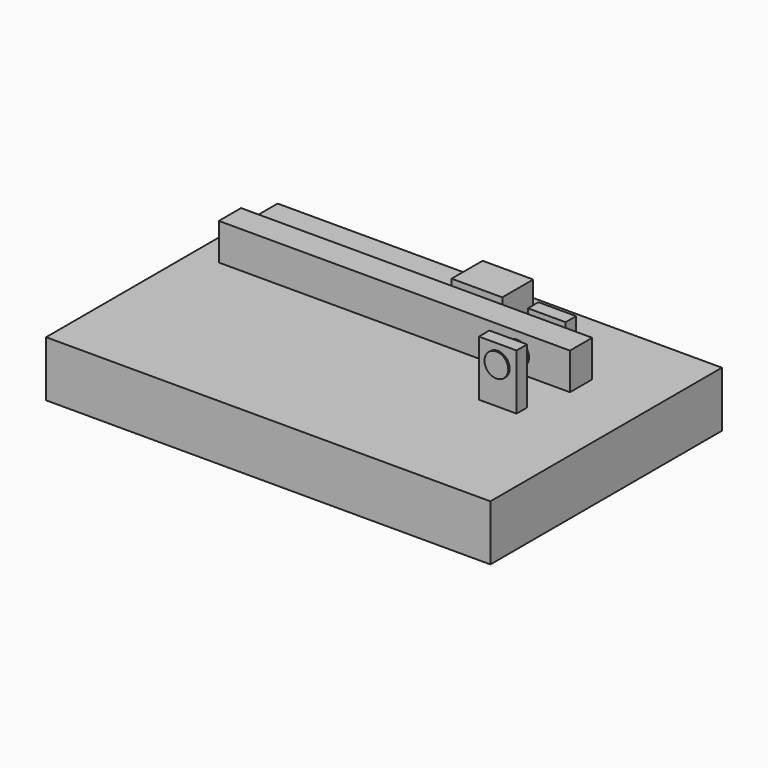
from build123d import *

# Parameters (mm, degrees)
F0_W      = 79.9336656928
F0_H      = 52.071608603
F1_DEPTH  = 10
F2_W      = 6.7777317017
F2_H      = 2.3667681962
F3_DEPTH  = 10
F6_R      = 2.1383442147
F7_DEPTH  = 7
F9_W      = 63.1709070876
F9_H      = 6.5956874751
F10_DEPTH = 2.5
F11_W     = 9.1101154685
F11_H     = 6.9677913561
F12_DEPTH = 10
F14_DEPTH = 2


# Not quite as in the source:
# - a feature of the source that left no trace in its solid (it failed there, or was rolled back) is left out


with BuildPart() as f1:
    # F0 (on Top) → F1 (new body)
    with BuildSketch(Plane.XY):
        with Locations((5.7745687664, -3.7935711443)):
            Rectangle(F0_W, F0_H)
    extrude(amount=-F1_DEPTH)


with BuildPart() as f3:
    # F2 (on face) → F3 (new body)
    with BuildSketch(Plane.XY):
        with Locations((28.5578714684, 5.5119483732)):
            Rectangle(F2_W, F2_H)
    extrude(amount=F3_DEPTH)


with BuildPart() as f3b:
    # F2 (on face) → F3, piece 2 (new body)
    with BuildSketch(Plane.XY):
        with Locations((28.5578714684, -5.5119483732)):
            Rectangle(F2_W, F2_H)
    extrude(amount=F3_DEPTH)


with BuildPart() as f7:
    # F6 (on Front) → F7 (new body, symmetric)
    with BuildSketch(Plane.XZ):
        with Locations((28.5583883524, 6.7135016434)):
            Circle(F6_R)
    extrude(amount=F7_DEPTH, both=True)


with BuildPart() as f10:
    # F9 (on offset) → F10 (new body, symmetric)
    with BuildSketch(Plane(origin=(0, 0.1714357249, 0), x_dir=(-1, 0, 0), z_dir=(0, 1, 0))):
        with Locations((-6.4699552022, 6.8944620434)):
            Rectangle(F9_W, F9_H)
    extrude(amount=F10_DEPTH, both=True)


with BuildPart() as f12:
    # F11 (on face) → F12 (new body)
    with BuildSketch(Plane.XY):
        with Locations((15.7252885401, 8.1531251781)):
            Rectangle(F11_W, F11_H)
    extrude(amount=F12_DEPTH)


with BuildPart() as f14:
    # F13 (on face) → F14 (new body)
    with BuildSketch(Plane.XZ.offset(-4.6692295)):
        with BuildLine():
            add(Edge.make_bspline(
                [(18.2029938622, 4.1400130684), (17.2900152833, 3.9210497766), (7.6229159122, 4.6514742458), (16.6876681251, 6.2329643074), (18.1721386483, 5.7793143696)],
                knots=[0, 0, 0, 0, 0.4111281062, 0.8221082471, 0.8221082471, 0.8221082471, 0.8221082471], degree=3))
            ThreePointArc((18.2029938622, 4.1400130684), (18.7000799562, 4.4130216349), (18.9044892921, 4.9420254964))
            add(Edge.make_bspline(
                [(18.1721386483, 5.7793143696), (18.8146880981, 5.5829530991), (18.8863438962, 5.1534723682), (18.9044892921, 4.9420254964)],
                knots=[0.8221082471, 0.8221082471, 0.8221082471, 0.8221082471, 1, 1, 1, 1], degree=3))
        make_face()
    extrude(amount=F14_DEPTH)


solid = Compound([f1.part, f3.part, f3b.part, f7.part, f10.part, f12.part, f14.part])
